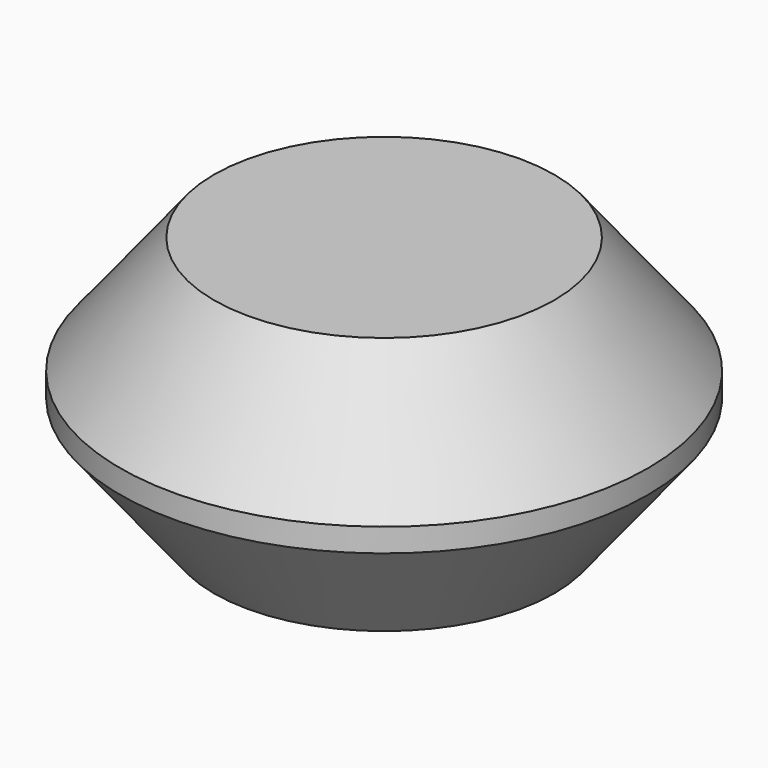
from build123d import *

# Parameters (mm, degrees)
F0_R      = 57.15
F1_DEPTH  = 2.54
F3_R      = 36.83
F1_FACE_R = 57.15


# Not quite as in the source:
# - the program builds the solid bodies; features that only make, move or delete a surface that nothing else refers to are left out


with BuildPart() as f1:
    # F0 (on Top) → F1 (new body)
    with BuildSketch(Plane.XY):
        Circle(F0_R)
    extrude(amount=F1_DEPTH)

    # F3 (on offset) → F4 section 0
    with BuildSketch(Plane.XY.offset(27.94)):
        Circle(F3_R)
    # F1_face (on face) → F4 section 1
    with BuildSketch(Plane.XY.offset(2.54)):
        Circle(F1_FACE_R)
    loft()

    # F5: F1 across face


with BuildPart() as f1_1:
    add(f1.part)
    add(f1.part.mirror(Plane(origin=(0, 0, 0), x_dir=(1, 0, 0), z_dir=(0, 0, -1))))


solid = f1_1.part
